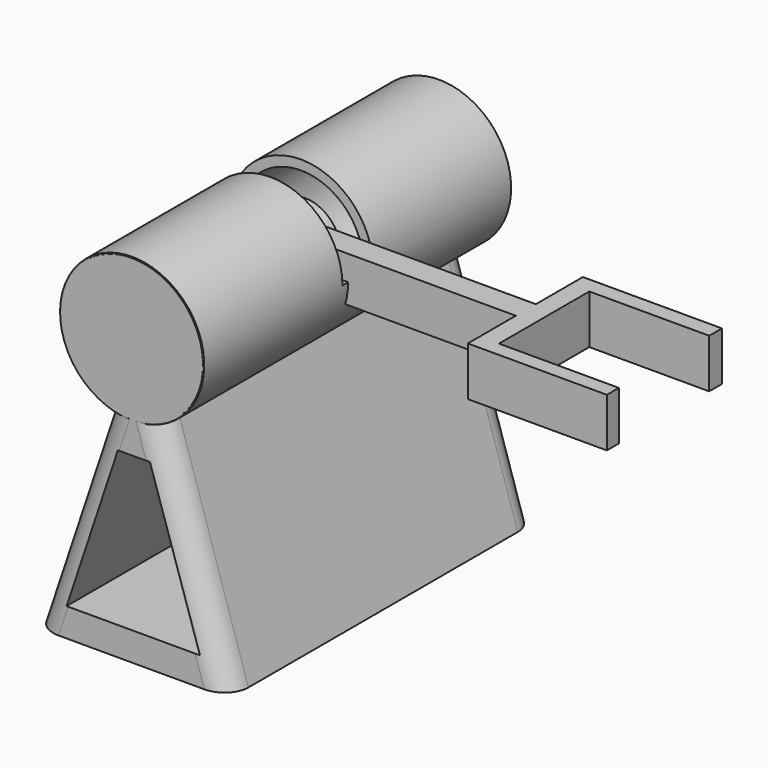
from build123d import *

# Parameters (mm, degrees)
F0_R          = 15.0415455236
F1_DEPTH      = 40
F2_R          = 13.0265097032
F3_DEPTH      = 80
F4_W          = 7.9495264217
F4_H          = 15.6480446458
F5_DEPTH      = 17.5
F6_R          = 7.5456912494
F7_DEPTH      = 5
F8_W          = 5.216877209
F8_H          = 9.4400634989
F9_DEPTH      = 50
F10_W         = 30
F10_H         = 10.2142902277
F11_DEPTH     = 4
F12_W         = 3.1286751479
F12_H         = 10.2142902277
F13_DEPTH     = 25
F14_W         = 3.3241308853
F14_H         = 10.2142902277
F15_DEPTH     = 25
F16_R         = 14.8524902499
F17_DEPTH     = 0.1
F18_R         = 14.6132587067
F19_DEPTH     = 0.1
F21_DEPTH     = 80.2
F23_DEPTH     = 80.201
F24_T4_DEPTH  = 73.2481904339
F24_S5_R      = 14.6132587067
F24_T6_DEPTH  = 40
F24_T11_DEPTH = 73.2481904339
F24_S12_R     = 15.0415455236
F24_T13_DEPTH = 40
F24_T17_DEPTH = 73.2835146544
F24_S18_R     = 15.0415455236
F24_T19_DEPTH = 40
F24_T23_DEPTH = 73.2835146544
F24_S24_R     = 14.6132587067
F24_T25_DEPTH = 40
F24_T30_DEPTH = 73.0440159481
F24_S31_R     = 15.0415455236
F24_T32_DEPTH = 40
F24_T36_DEPTH = 73.0440159481
F24_S37_R     = 14.8524902499
F24_T38_DEPTH = 40
F24_T43_DEPTH = 73.0079978677
F24_S44_R     = 14.8524902499
F24_T45_DEPTH = 40
F24_T50_DEPTH = 73.0079978677
F24_S51_R     = 15.0415455236
F24_T52_DEPTH = 40


# Not quite as in the source:
# - a fillet or chamfer that OpenCascade refuses, or shapes differently, is made with other operations: its cross-section is extruded or revolved along the edge and cut away or added


with BuildPart() as f1:
    # F0 (on Front) → F1 (new body, symmetric)
    with BuildSketch(Plane.XZ):
        Circle(F0_R)
    extrude(amount=F1_DEPTH, both=True)

    # F2 (on face) → F3 (cut)
    with BuildSketch(Plane.XZ.offset(40)):
        Circle(F2_R)
    extrude(amount=-F3_DEPTH, mode=Mode.SUBTRACT)

    # F4 (on Right) → F5 (cut, symmetric)
    with BuildSketch(Plane.YZ):
        with Locations((0, 7.8240223229)):
            Rectangle(F4_W, F4_H)
    extrude(amount=F5_DEPTH, both=True, mode=Mode.SUBTRACT)

    # F16 (on face) → F17 (join)
    with BuildSketch(Plane.XZ.offset(40)):
        Circle(F16_R)
    extrude(amount=F17_DEPTH)

    # F18 (on face) → F19 (join)
    with BuildSketch(Plane(origin=(0, 40, 0), x_dir=(-1, 0, 0), z_dir=(0, 1, 0))):
        Circle(F18_R)
    extrude(amount=F19_DEPTH)

    # F20 (on face) → F21 (join)
    with BuildSketch(Plane(origin=(0, 40.1, 0), x_dir=(-1, 0, 0), z_dir=(0, 1, 0))):
        Polygon((5.2737725107, -13.6284501516), (-5.6739483665, -13.4667605594), (-20.3254725784, -59.4365410507), (20.5353777856, -59.4365410507), align=None)
    extrude(amount=-F21_DEPTH)

    # F22 (on face) → F23 (cut, through all)
    with BuildSketch(Plane.XZ.offset(40.1)):
        Polygon((-2.9082546706, -21.3973574286), (-13.6014148593, -53.4931458533), (14.1344349831, -53.4931458533), (3.7334910594, -21.3973574286), align=None)
    extrude(amount=-F23_DEPTH, mode=Mode.SUBTRACT)

    # F24: fillet of radius 5 on 4 edges, made by hand


with BuildPart() as f7:
    # F6 (on Front) → F7 (new body, symmetric)
    with BuildSketch(Plane.XZ):
        Circle(F6_R)
    extrude(amount=F7_DEPTH, both=True)

    # F8 (on Right) → F9 (join)
    with BuildSketch(Plane.YZ):
        with Locations((0.1242113067, 0.4942584783)):
            Rectangle(F8_W, F8_H)
    extrude(amount=F9_DEPTH)

    # F10 (on face) → F11 (join)
    with BuildSketch(Plane.YZ.offset(50)):
        with Locations((0, 0.1071451139)):
            Rectangle(F10_W, F10_H)
    extrude(amount=F11_DEPTH)

    # F12 (on face) → F13 (join)
    with BuildSketch(Plane.YZ.offset(54)):
        with Locations((-13.4356624261, 0.1071451139)):
            Rectangle(F12_W, F12_H)
    extrude(amount=F13_DEPTH)

    # F14 (on face) → F15 (join)
    with BuildSketch(Plane.YZ.offset(54)):
        with Locations((13.3379345573, 0.1071451139)):
            Rectangle(F14_W, F14_H)
    extrude(amount=F15_DEPTH)


with BuildPart() as f24_tool2:
    # F24_s3 → F24_t4 (new body)
    with BuildSketch(Plane(origin=(0.6236867561, 0, -1.9568437291), x_dir=(0, 1, 0), z_dir=(0.3036699217, 0, -0.9527772975))):
        with BuildLine():
            ThreePointArc((35.1, 1.3165590661), (38.6355339059, -0.147907028), (40.1, -3.6834409339))
            Line((40.1, -3.6834409339), (40.1, 1.3165590661))
            Line((40.1, 1.3165590661), (35.1, 1.3165590661))
        make_face()
    extrude(amount=F24_T4_DEPTH)

    # F24_s5 → F24_t6 (cut, symmetric)
    with BuildSketch(Plane.XZ.offset(-37.6)):
        Circle(F24_S5_R)
    extrude(amount=F24_T6_DEPTH, both=True, mode=Mode.SUBTRACT)

    split(bisect_by=Plane.XZ.offset(-40), keep=Keep.BOTTOM)


with BuildPart() as f1_1:
    add(f1.part)

    # F24_t1: cut F24_tool2
    add(f24_tool2.part, mode=Mode.SUBTRACT)


with BuildPart() as f24_tool9:
    # F24_s10 → F24_t11 (new body)
    with BuildSketch(Plane(origin=(0.6236867561, 0, -1.9568437291), x_dir=(0, 1, 0), z_dir=(0.3036699217, 0, -0.9527772975))):
        with BuildLine():
            ThreePointArc((35.1, 1.3165590661), (38.6355339059, -0.147907028), (40.1, -3.6834409339))
            Line((40.1, -3.6834409339), (40.1, 1.3165590661))
            Line((40.1, 1.3165590661), (35.1, 1.3165590661))
        make_face()
    extrude(amount=F24_T11_DEPTH)

    # F24_s12 → F24_t13 (cut, symmetric)
    with BuildSketch(Plane.XZ.offset(-37.6)):
        Circle(F24_S12_R)
    extrude(amount=F24_T13_DEPTH, both=True, mode=Mode.SUBTRACT)


with BuildPart() as f1_2:
    add(f1_1.part)

    # F24_t8: cut F24_tool9
    add(f24_tool9.part, mode=Mode.SUBTRACT)


with BuildPart() as f24_tool15:
    # F24_s16 → F24_t17 (new body)
    with BuildSketch(Plane(origin=(-23.8264124769, 0, -71.5155744685), x_dir=(0, 1, 0), z_dir=(0.3160831473, 0, 0.948731492))):
        with BuildLine():
            ThreePointArc((35.1, 0.695670646), (38.6355339059, -0.7687954481), (40.1, -4.304329354))
            Line((40.1, -4.304329354), (40.1, 0.695670646))
            Line((40.1, 0.695670646), (35.1, 0.695670646))
        make_face()
    extrude(amount=F24_T17_DEPTH)

    # F24_s18 → F24_t19 (cut, symmetric)
    with BuildSketch(Plane.XZ.offset(-37.6)):
        Circle(F24_S18_R)
    extrude(amount=F24_T19_DEPTH, both=True, mode=Mode.SUBTRACT)


with BuildPart() as f1_3:
    add(f1_2.part)

    # F24_t14: cut F24_tool15
    add(f24_tool15.part, mode=Mode.SUBTRACT)


with BuildPart() as f24_tool21:
    # F24_s22 → F24_t23 (new body)
    with BuildSketch(Plane(origin=(-23.8264124769, 0, -71.5155744685), x_dir=(0, 1, 0), z_dir=(0.3160831473, 0, 0.948731492))):
        with BuildLine():
            ThreePointArc((35.1, 0.695670646), (38.6355339059, -0.7687954481), (40.1, -4.304329354))
            Line((40.1, -4.304329354), (40.1, 0.695670646))
            Line((40.1, 0.695670646), (35.1, 0.695670646))
        make_face()
    extrude(amount=F24_T23_DEPTH)

    # F24_s24 → F24_t25 (cut, symmetric)
    with BuildSketch(Plane.XZ.offset(-37.6)):
        Circle(F24_S24_R)
    extrude(amount=F24_T25_DEPTH, both=True, mode=Mode.SUBTRACT)

    split(bisect_by=Plane.XZ.offset(-40), keep=Keep.BOTTOM)


with BuildPart() as f1_4:
    add(f1_3.part)

    # F24_t20: cut F24_tool21
    add(f24_tool21.part, mode=Mode.SUBTRACT)


with BuildPart() as f24_tool28:
    # F24_s29 → F24_t30 (new body)
    with BuildSketch(Plane(origin=(-23.8264124769, 0, -71.5155744685), x_dir=(0, 1, 0), z_dir=(0.3160831473, 0, 0.948731492))):
        with BuildLine():
            ThreePointArc((-35.1, 0.695670646), (-38.6355339059, -0.7687954481), (-40.1, -4.304329354))
            Line((-40.1, -4.304329354), (-40.1, 0.695670646))
            Line((-40.1, 0.695670646), (-35.1, 0.695670646))
        make_face()
    extrude(amount=F24_T30_DEPTH)

    # F24_s31 → F24_t32 (cut, symmetric)
    with BuildSketch(Plane.XZ.offset(37.6)):
        Circle(F24_S31_R)
    extrude(amount=F24_T32_DEPTH, both=True, mode=Mode.SUBTRACT)


with BuildPart() as f1_5:
    add(f1_4.part)

    # F24_t27: cut F24_tool28
    add(f24_tool28.part, mode=Mode.SUBTRACT)


with BuildPart() as f24_tool34:
    # F24_s35 → F24_t36 (new body)
    with BuildSketch(Plane(origin=(-23.8264124769, 0, -71.5155744685), x_dir=(0, 1, 0), z_dir=(0.3160831473, 0, 0.948731492))):
        with BuildLine():
            ThreePointArc((-35.1, 0.695670646), (-38.6355339059, -0.7687954481), (-40.1, -4.304329354))
            Line((-40.1, -4.304329354), (-40.1, 0.695670646))
            Line((-40.1, 0.695670646), (-35.1, 0.695670646))
        make_face()
    extrude(amount=F24_T36_DEPTH)

    # F24_s37 → F24_t38 (cut, symmetric)
    with BuildSketch(Plane.XZ.offset(37.6)):
        Circle(F24_S37_R)
    extrude(amount=F24_T38_DEPTH, both=True, mode=Mode.SUBTRACT)

    split(bisect_by=Plane.XZ.offset(40), keep=Keep.TOP)


with BuildPart() as f1_6:
    add(f1_5.part)

    # F24_t33: cut F24_tool34
    add(f24_tool34.part, mode=Mode.SUBTRACT)


with BuildPart() as f24_tool41:
    # F24_s42 → F24_t43 (new body)
    with BuildSketch(Plane(origin=(0.6966260139, 0, -2.1856937532), x_dir=(0, 1, 0), z_dir=(0.3036699217, 0, -0.9527772975))):
        with BuildLine():
            ThreePointArc((-35.1, 1.3165590661), (-38.6355339059, -0.147907028), (-40.1, -3.6834409339))
            Line((-40.1, -3.6834409339), (-40.1, 1.3165590661))
            Line((-40.1, 1.3165590661), (-35.1, 1.3165590661))
        make_face()
    extrude(amount=F24_T43_DEPTH)

    # F24_s44 → F24_t45 (cut, symmetric)
    with BuildSketch(Plane.XZ.offset(37.6)):
        Circle(F24_S44_R)
    extrude(amount=F24_T45_DEPTH, both=True, mode=Mode.SUBTRACT)

    split(bisect_by=Plane.XZ.offset(40), keep=Keep.TOP)


with BuildPart() as f1_7:
    add(f1_6.part)

    # F24_t40: cut F24_tool41
    add(f24_tool41.part, mode=Mode.SUBTRACT)


with BuildPart() as f24_tool48:
    # F24_s49 → F24_t50 (new body)
    with BuildSketch(Plane(origin=(0.6966260139, 0, -2.1856937532), x_dir=(0, 1, 0), z_dir=(0.3036699217, 0, -0.9527772975))):
        with BuildLine():
            ThreePointArc((-35.1, 1.3165590661), (-38.6355339059, -0.147907028), (-40.1, -3.6834409339))
            Line((-40.1, -3.6834409339), (-40.1, 1.3165590661))
            Line((-40.1, 1.3165590661), (-35.1, 1.3165590661))
        make_face()
    extrude(amount=F24_T50_DEPTH)

    # F24_s51 → F24_t52 (cut, symmetric)
    with BuildSketch(Plane.XZ.offset(37.6)):
        Circle(F24_S51_R)
    extrude(amount=F24_T52_DEPTH, both=True, mode=Mode.SUBTRACT)


with BuildPart() as f1_8:
    add(f1_7.part)

    # F24_t47: cut F24_tool48
    add(f24_tool48.part, mode=Mode.SUBTRACT)


solid = Compound([f7.part, f1_8.part])
